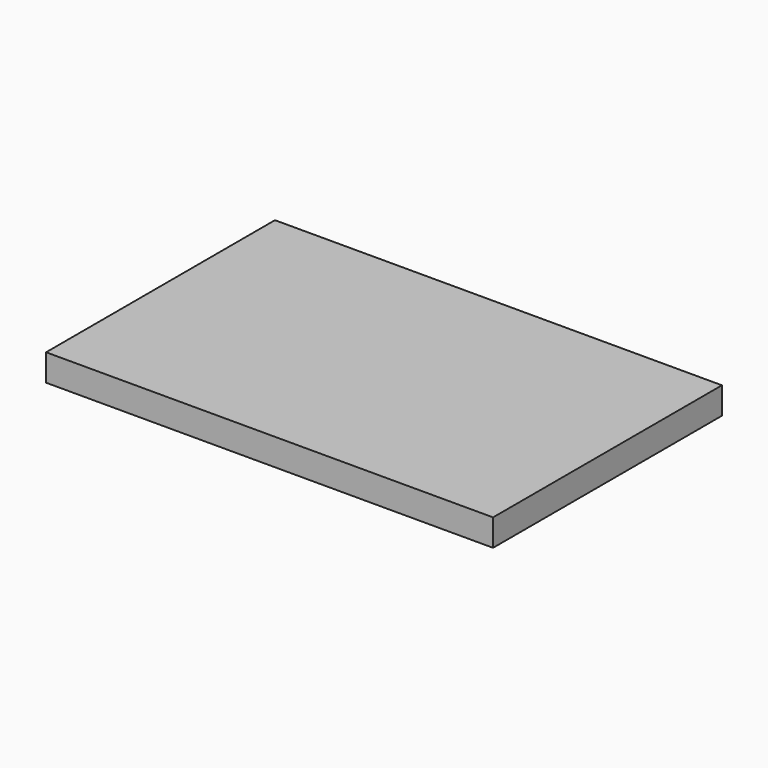
from build123d import *

# Parameters (mm, degrees)
F0_W     = 158.75
F0_H     = 101.6
F1_DEPTH = 9.525


# Not quite as in the source:
# - a length typed as a fraction of an inch, garbled in the dataset ("3 / 203.2 mm" for 3/8 in), is restored


with BuildPart() as f1:
    # F0 (on Top) → F1 (new body)
    with BuildSketch(Plane.XY):
        Rectangle(F0_W, F0_H)
    extrude(amount=F1_DEPTH)


solid = f1.part
